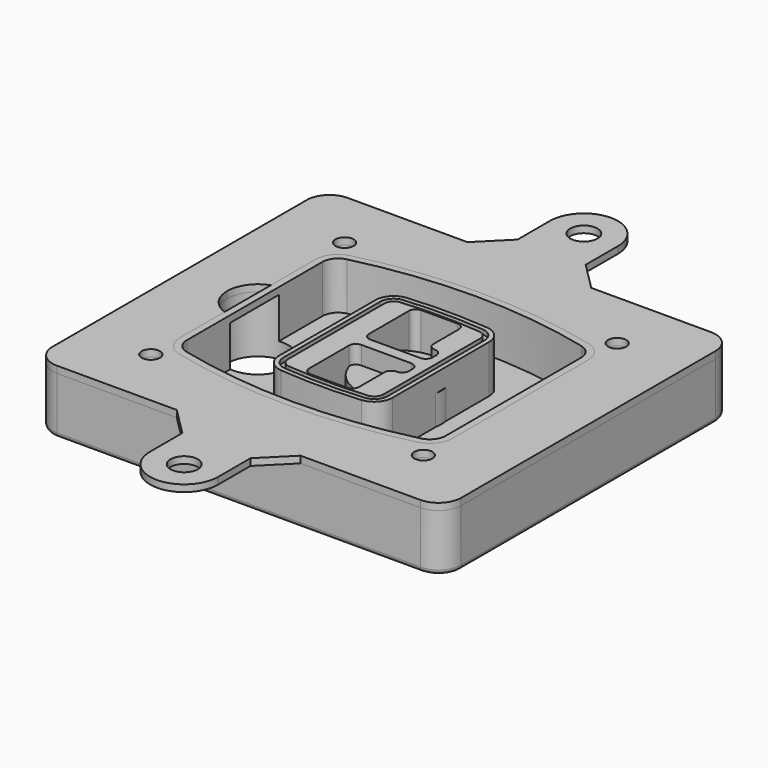
from build123d import *

# Parameters (mm, degrees)
F0_R      = 4
F1_DEPTH  = 25
F2_DEPTH  = 3
F3_DEPTH  = 18
F5_DEPTH  = 21
F6_DEPTH  = 2
F8_DEPTH  = 20
F9_DEPTH  = 16
F10_DEPTH = 25
F7_R      = 6
F7_R_2    = 4
F11_DEPTH = 6
F13_DEPTH = 9
F15_R     = 2
F16_R     = 6
F16_R_2   = 4
F17_DEPTH = 3


# Not quite as in the source:
# - a feature of the source that left no trace in its solid (it failed there, or was rolled back) is left out
# - a feature names something its author has since deleted; it is built from what else it names


with BuildPart() as f1:
    # F0 (on Top) → F1 (new body)
    with BuildSketch(Plane.XY):
        with BuildLine():
            ThreePointArc((-90, -70), (-87.0710678119, -77.0710678119), (-80, -80))
            Line((-80, -80), (80, -80))
            ThreePointArc((80, -80), (87.0710678119, -77.0710678119), (90, -70))
            Line((90, -70), (90, 70))
            ThreePointArc((90, 70), (87.0710678119, 77.0710678119), (80, 80))
            Line((80, 80), (-80, 80))
            ThreePointArc((-80, 80), (-87.0710678119, 77.0710678119), (-90, 70))
            Line((-90, 70), (-90, -70))
        make_face()
        with Locations((-60, -53.3333333333)):
            Circle(F0_R, mode=Mode.SUBTRACT)
        with Locations((60, -53.3333333333)):
            Circle(F0_R, mode=Mode.SUBTRACT)
        with Locations((-60, 53.3333333333)):
            Circle(F0_R, mode=Mode.SUBTRACT)
        with BuildLine():
            ThreePointArc((-64, 37.2990447398), (-61.0143011354, 45.9411029726), (-53.3306899286, 50.8970778549))
            ThreePointArc((-53.3306899286, 50.8970778549), (0, 57.3333333333), (53.3306899286, 50.8970778549))
            ThreePointArc((53.3306899286, 50.8970778549), (61.0143011354, 45.9411029726), (64, 37.2990447398))
            Line((64, 37.2990447398), (64, -37.2990447398))
            ThreePointArc((64, -37.2990447398), (61.0143011354, -45.9411029726), (53.3306899286, -50.8970778549))
            ThreePointArc((53.3306899286, -50.8970778549), (0, -57.3333333333), (-53.3306899286, -50.8970778549))
            ThreePointArc((-53.3306899286, -50.8970778549), (-61.0143011354, -45.9411029726), (-64, -37.2990447398))
            Line((-64, -37.2990447398), (-64, 37.2990447398))
        make_face(mode=Mode.SUBTRACT)
        with Locations((60, 53.3333333333)):
            Circle(F0_R, mode=Mode.SUBTRACT)
        with BuildLine():
            ThreePointArc((53.3306899286, 50.8970778549), (0, 57.3333333333), (-53.3306899286, 50.8970778549))
            ThreePointArc((-53.3306899286, 50.8970778549), (-61.0143011354, 45.9411029726), (-64, 37.2990447398))
            Line((-64, 37.2990447398), (-64, -37.2990447398))
            ThreePointArc((-64, -37.2990447398), (-61.0143011354, -45.9411029726), (-53.3306899286, -50.8970778549))
            ThreePointArc((-53.3306899286, -50.8970778549), (0, -57.3333333333), (53.3306899286, -50.8970778549))
            ThreePointArc((53.3306899286, -50.8970778549), (61.0143011354, -45.9411029726), (64, -37.2990447398))
            Line((64, -37.2990447398), (64, 37.2990447398))
            ThreePointArc((64, 37.2990447398), (61.0143011354, 45.9411029726), (53.3306899286, 50.8970778549))
        make_face()
        with BuildLine():
            Line((-60, -37.2990447398), (-60, 37.2990447398))
            ThreePointArc((-60, 37.2990447398), (-57.8673579538, 43.4719434775), (-52.3790642347, 47.0119255363))
            ThreePointArc((-52.3790642347, 47.0119255363), (0, 53.3333333333), (52.3790642347, 47.0119255363))
            ThreePointArc((52.3790642347, 47.0119255363), (57.8673579538, 43.4719434775), (60, 37.2990447398))
            Line((60, 37.2990447398), (60, -37.2990447398))
            ThreePointArc((60, -37.2990447398), (57.8673579538, -43.4719434775), (52.3790642347, -47.0119255363))
            ThreePointArc((52.3790642347, -47.0119255363), (0, -53.3333333333), (-52.3790642347, -47.0119255363))
            ThreePointArc((-52.3790642347, -47.0119255363), (-57.8673579538, -43.4719434775), (-60, -37.2990447398))
        make_face(mode=Mode.SUBTRACT)
        with BuildLine():
            ThreePointArc((-52.3790642347, 47.0119255363), (-57.8673579538, 43.4719434775), (-60, 37.2990447398))
            Line((-60, 37.2990447398), (-60, -37.2990447398))
            ThreePointArc((-60, -37.2990447398), (-57.8673579538, -43.4719434775), (-52.3790642347, -47.0119255363))
            ThreePointArc((-52.3790642347, -47.0119255363), (0, -53.3333333333), (52.3790642347, -47.0119255363))
            ThreePointArc((52.3790642347, -47.0119255363), (57.8673579538, -43.4719434775), (60, -37.2990447398))
            Line((60, -37.2990447398), (60, 37.2990447398))
            ThreePointArc((60, 37.2990447398), (57.8673579538, 43.4719434775), (52.3790642347, 47.0119255363))
            ThreePointArc((52.3790642347, 47.0119255363), (0, 53.3333333333), (-52.3790642347, 47.0119255363))
        make_face()
        with BuildLine():
            ThreePointArc((51.6653449643, 44.0980612973), (55.5071505677, 41.6200738562), (57, 37.2990447398))
            Line((57, 37.2990447398), (57, -37.2990447398))
            ThreePointArc((57, -37.2990447398), (55.5071505677, -41.6200738562), (51.6653449643, -44.0980612973))
            ThreePointArc((51.6653449643, -44.0980612973), (0, -50.3333333333), (-51.6653449643, -44.0980612973))
            ThreePointArc((-51.6653449643, -44.0980612973), (-55.5071505677, -41.6200738562), (-57, -37.2990447398))
            Line((-57, -37.2990447398), (-57, 37.2990447398))
            ThreePointArc((-57, 37.2990447398), (-55.5071505677, 41.6200738562), (-51.6653449643, 44.0980612973))
            ThreePointArc((-51.6653449643, 44.0980612973), (0, 50.3333333333), (51.6653449643, 44.0980612973))
        make_face(mode=Mode.SUBTRACT)
        with BuildLine():
            Line((57, -37.2990447398), (57, 37.2990447398))
            ThreePointArc((57, 37.2990447398), (55.5071505677, 41.6200738562), (51.6653449643, 44.0980612973))
            ThreePointArc((51.6653449643, 44.0980612973), (0, 50.3333333333), (-51.6653449643, 44.0980612973))
            ThreePointArc((-51.6653449643, 44.0980612973), (-55.5071505677, 41.6200738562), (-57, 37.2990447398))
            Line((-57, 37.2990447398), (-57, -37.2990447398))
            ThreePointArc((-57, -37.2990447398), (-55.5071505677, -41.6200738562), (-51.6653449643, -44.0980612973))
            ThreePointArc((-51.6653449643, -44.0980612973), (0, -50.3333333333), (51.6653449643, -44.0980612973))
            ThreePointArc((51.6653449643, -44.0980612973), (55.5071505677, -41.6200738562), (57, -37.2990447398))
        make_face()
    extrude(amount=-F1_DEPTH)

    # F0 (on Top) → F2 (join)
    with BuildSketch(Plane.XY):
        with BuildLine():
            ThreePointArc((-52.3790642347, 47.0119255363), (-57.8673579538, 43.4719434775), (-60, 37.2990447398))
            Line((-60, 37.2990447398), (-60, -37.2990447398))
            ThreePointArc((-60, -37.2990447398), (-57.8673579538, -43.4719434775), (-52.3790642347, -47.0119255363))
            ThreePointArc((-52.3790642347, -47.0119255363), (0, -53.3333333333), (52.3790642347, -47.0119255363))
            ThreePointArc((52.3790642347, -47.0119255363), (57.8673579538, -43.4719434775), (60, -37.2990447398))
            Line((60, -37.2990447398), (60, 37.2990447398))
            ThreePointArc((60, 37.2990447398), (57.8673579538, 43.4719434775), (52.3790642347, 47.0119255363))
            ThreePointArc((52.3790642347, 47.0119255363), (0, 53.3333333333), (-52.3790642347, 47.0119255363))
        make_face()
        with BuildLine():
            ThreePointArc((51.6653449643, 44.0980612973), (55.5071505677, 41.6200738562), (57, 37.2990447398))
            Line((57, 37.2990447398), (57, -37.2990447398))
            ThreePointArc((57, -37.2990447398), (55.5071505677, -41.6200738562), (51.6653449643, -44.0980612973))
            ThreePointArc((51.6653449643, -44.0980612973), (0, -50.3333333333), (-51.6653449643, -44.0980612973))
            ThreePointArc((-51.6653449643, -44.0980612973), (-55.5071505677, -41.6200738562), (-57, -37.2990447398))
            Line((-57, -37.2990447398), (-57, 37.2990447398))
            ThreePointArc((-57, 37.2990447398), (-55.5071505677, 41.6200738562), (-51.6653449643, 44.0980612973))
            ThreePointArc((-51.6653449643, 44.0980612973), (0, 50.3333333333), (51.6653449643, 44.0980612973))
        make_face(mode=Mode.SUBTRACT)
    extrude(amount=F2_DEPTH)

    # F0 (on Top) → F3 (cut)
    with BuildSketch(Plane.XY):
        with BuildLine():
            Line((57, -37.2990447398), (57, 37.2990447398))
            ThreePointArc((57, 37.2990447398), (55.5071505677, 41.6200738562), (51.6653449643, 44.0980612973))
            ThreePointArc((51.6653449643, 44.0980612973), (0, 50.3333333333), (-51.6653449643, 44.0980612973))
            ThreePointArc((-51.6653449643, 44.0980612973), (-55.5071505677, 41.6200738562), (-57, 37.2990447398))
            Line((-57, 37.2990447398), (-57, -37.2990447398))
            ThreePointArc((-57, -37.2990447398), (-55.5071505677, -41.6200738562), (-51.6653449643, -44.0980612973))
            ThreePointArc((-51.6653449643, -44.0980612973), (0, -50.3333333333), (51.6653449643, -44.0980612973))
            ThreePointArc((51.6653449643, -44.0980612973), (55.5071505677, -41.6200738562), (57, -37.2990447398))
        make_face()
    extrude(amount=-F3_DEPTH, mode=Mode.SUBTRACT)

    # F4 (on face) → F5 (join, through all)
    with BuildSketch(Plane.XY.offset(3)):
        with BuildLine():
            ThreePointArc((-25, -26.587695628), (-22.8992979869, -31.9912392117), (-17.7004291845, -34.5569740744))
            ThreePointArc((-17.7004291845, -34.5569740744), (0, -35.3333333333), (17.7004291845, -34.5569740744))
            ThreePointArc((17.7004291845, -34.5569740744), (22.8992979869, -31.9912392117), (25, -26.587695628))
            Line((25, -26.587695628), (25, 26.587695628))
            ThreePointArc((25, 26.587695628), (22.8992979869, 31.9912392117), (17.7004291845, 34.5569740744))
            ThreePointArc((17.7004291845, 34.5569740744), (0, 35.3333333333), (-17.7004291845, 34.5569740744))
            ThreePointArc((-17.7004291845, 34.5569740744), (-22.8992979869, 31.9912392117), (-25, 26.587695628))
            Line((-25, 26.587695628), (-25, -26.587695628))
        make_face()
        with BuildLine():
            ThreePointArc((17.5253218884, 32.5646544628), (21.4244734902, 30.6403533158), (23, 26.587695628))
            Line((23, 26.587695628), (23, -26.587695628))
            ThreePointArc((23, -26.587695628), (21.4244734902, -30.6403533158), (17.5253218884, -32.5646544628))
            ThreePointArc((17.5253218884, -32.5646544628), (0, -33.3333333333), (-17.5253218884, -32.5646544628))
            ThreePointArc((-17.5253218884, -32.5646544628), (-21.4244734902, -30.6403533158), (-23, -26.587695628))
            Line((-23, -26.587695628), (-23, 26.587695628))
            ThreePointArc((-23, 26.587695628), (-21.4244734902, 30.6403533158), (-17.5253218884, 32.5646544628))
            ThreePointArc((-17.5253218884, 32.5646544628), (0, 33.3333333333), (17.5253218884, 32.5646544628))
        make_face(mode=Mode.SUBTRACT)
        with BuildLine():
            Line((23, -26.587695628), (23, 26.587695628))
            ThreePointArc((23, 26.587695628), (21.4244734902, 30.6403533158), (17.5253218884, 32.5646544628))
            ThreePointArc((17.5253218884, 32.5646544628), (0, 33.3333333333), (-17.5253218884, 32.5646544628))
            ThreePointArc((-17.5253218884, 32.5646544628), (-21.4244734902, 30.6403533158), (-23, 26.587695628))
            Line((-23, 26.587695628), (-23, -26.587695628))
            ThreePointArc((-23, -26.587695628), (-21.4244734902, -30.6403533158), (-17.5253218884, -32.5646544628))
            ThreePointArc((-17.5253218884, -32.5646544628), (0, -33.3333333333), (17.5253218884, -32.5646544628))
            ThreePointArc((17.5253218884, -32.5646544628), (21.4244734902, -30.6403533158), (23, -26.587695628))
        make_face()
        with BuildLine():
            ThreePointArc((17.3502145923, 30.5723348512), (19.9496489934, 29.2894674198), (21, 26.587695628))
            Line((21, 26.587695628), (21, -26.587695628))
            ThreePointArc((21, -26.587695628), (19.9496489934, -29.2894674198), (17.3502145923, -30.5723348512))
            ThreePointArc((17.3502145923, -30.5723348512), (0, -31.3333333333), (-17.3502145923, -30.5723348512))
            ThreePointArc((-17.3502145923, -30.5723348512), (-19.9496489934, -29.2894674198), (-21, -26.587695628))
            Line((-21, -26.587695628), (-21, 26.587695628))
            ThreePointArc((-21, 26.587695628), (-19.9496489934, 29.2894674198), (-17.3502145923, 30.5723348512))
            ThreePointArc((-17.3502145923, 30.5723348512), (0, 31.3333333333), (17.3502145923, 30.5723348512))
        make_face(mode=Mode.SUBTRACT)
        with BuildLine():
            Line((21, -26.587695628), (21, 26.587695628))
            ThreePointArc((21, 26.587695628), (19.9496489934, 29.2894674198), (17.3502145923, 30.5723348512))
            ThreePointArc((17.3502145923, 30.5723348512), (0, 31.3333333333), (-17.3502145923, 30.5723348512))
            ThreePointArc((-17.3502145923, 30.5723348512), (-19.9496489934, 29.2894674198), (-21, 26.587695628))
            Line((-21, 26.587695628), (-21, -26.587695628))
            ThreePointArc((-21, -26.587695628), (-19.9496489934, -29.2894674198), (-17.3502145923, -30.5723348512))
            ThreePointArc((-17.3502145923, -30.5723348512), (0, -31.3333333333), (17.3502145923, -30.5723348512))
            ThreePointArc((17.3502145923, -30.5723348512), (19.9496489934, -29.2894674198), (21, -26.587695628))
        make_face()
        with BuildLine():
            Line((-8, -2.5), (14, -2.5))
            ThreePointArc((14, -2.5), (16.1213203436, -3.3786796564), (17, -5.5))
            Line((17, -5.5), (17, -7.5))
            ThreePointArc((17, -7.5), (16.1213203436, -9.6213203436), (14, -10.5))
            ThreePointArc((14, -10.5), (11.8786796564, -11.3786796564), (11, -13.5))
            Line((11, -13.5), (11, -27.5))
            ThreePointArc((11, -27.5), (10.1213203436, -29.6213203436), (8, -30.5))
            Line((8, -30.5), (-8, -30.5))
            ThreePointArc((-8, -30.5), (-10.1213203436, -29.6213203436), (-11, -27.5))
            Line((-11, -27.5), (-11, -5.5))
            ThreePointArc((-11, -5.5), (-10.1213203436, -3.3786796564), (-8, -2.5))
        make_face(mode=Mode.SUBTRACT)
        with BuildLine():
            ThreePointArc((-8, 2.5), (-10.1213203436, 3.3786796564), (-11, 5.5))
            Line((-11, 5.5), (-11, 27.5))
            ThreePointArc((-11, 27.5), (-10.1213203436, 29.6213203436), (-8, 30.5))
            Line((-8, 30.5), (8, 30.5))
            ThreePointArc((8, 30.5), (10.1213203436, 29.6213203436), (11, 27.5))
            Line((11, 27.5), (11, 13.5))
            ThreePointArc((11, 13.5), (11.8786796564, 11.3786796564), (14, 10.5))
            ThreePointArc((14, 10.5), (16.1213203436, 9.6213203436), (17, 7.5))
            Line((17, 7.5), (17, 5.5))
            ThreePointArc((17, 5.5), (16.1213203436, 3.3786796564), (14, 2.5))
            Line((14, 2.5), (-8, 2.5))
        make_face(mode=Mode.SUBTRACT)
    extrude(amount=-F5_DEPTH)

    # F4 (on face) → F6 (cut)
    with BuildSketch(Plane.XY.offset(3)):
        with BuildLine():
            Line((23, -26.587695628), (23, 26.587695628))
            ThreePointArc((23, 26.587695628), (21.4244734902, 30.6403533158), (17.5253218884, 32.5646544628))
            ThreePointArc((17.5253218884, 32.5646544628), (0, 33.3333333333), (-17.5253218884, 32.5646544628))
            ThreePointArc((-17.5253218884, 32.5646544628), (-21.4244734902, 30.6403533158), (-23, 26.587695628))
            Line((-23, 26.587695628), (-23, -26.587695628))
            ThreePointArc((-23, -26.587695628), (-21.4244734902, -30.6403533158), (-17.5253218884, -32.5646544628))
            ThreePointArc((-17.5253218884, -32.5646544628), (0, -33.3333333333), (17.5253218884, -32.5646544628))
            ThreePointArc((17.5253218884, -32.5646544628), (21.4244734902, -30.6403533158), (23, -26.587695628))
        make_face()
        with BuildLine():
            ThreePointArc((17.3502145923, 30.5723348512), (19.9496489934, 29.2894674198), (21, 26.587695628))
            Line((21, 26.587695628), (21, -26.587695628))
            ThreePointArc((21, -26.587695628), (19.9496489934, -29.2894674198), (17.3502145923, -30.5723348512))
            ThreePointArc((17.3502145923, -30.5723348512), (0, -31.3333333333), (-17.3502145923, -30.5723348512))
            ThreePointArc((-17.3502145923, -30.5723348512), (-19.9496489934, -29.2894674198), (-21, -26.587695628))
            Line((-21, -26.587695628), (-21, 26.587695628))
            ThreePointArc((-21, 26.587695628), (-19.9496489934, 29.2894674198), (-17.3502145923, 30.5723348512))
            ThreePointArc((-17.3502145923, 30.5723348512), (0, 31.3333333333), (17.3502145923, 30.5723348512))
        make_face(mode=Mode.SUBTRACT)
    extrude(amount=-F6_DEPTH, mode=Mode.SUBTRACT)

    # F7 (on face) → F8 (join)
    with BuildSketch(Plane(origin=(0, 0, -25), x_dir=(1, 0, 0), z_dir=(0, 0, -1))):
        with BuildLine():
            ThreePointArc((-6.71157564, 0), (6.7567035675, 13.4682792075), (20.224982775, 0))
            Line((20.224982775, 0), (25.224982775, 0))
            ThreePointArc((25.224982775, 0), (6.7567035675, 18.4682792075), (-11.71157564, 0))
            Line((-11.71157564, 0), (-6.71157564, 0))
        make_face()
        with BuildLine():
            Line((-6.71157564, 0), (20.224982775, 0))
            ThreePointArc((20.224982775, 0), (6.7567035675, 13.4682792075), (-6.71157564, 0))
        make_face()
        with BuildLine():
            ThreePointArc((-6.71157564, 0), (6.7567035675, -13.4682792075), (20.224982775, 0))
            Line((20.224982775, 0), (-6.71157564, 0))
        make_face()
        with BuildLine():
            Line((25.224982775, 0), (20.224982775, 0))
            ThreePointArc((20.224982775, 0), (6.7567035675, -13.4682792075), (-6.71157564, 0))
            Line((-6.71157564, 0), (-11.71157564, 0))
            ThreePointArc((-11.71157564, 0), (6.7567035675, -18.4682792075), (25.224982775, 0))
        make_face()
    extrude(amount=-F8_DEPTH)

    # F7 (on face) → F9 (cut)
    with BuildSketch(Plane(origin=(0, 0, -25), x_dir=(1, 0, 0), z_dir=(0, 0, -1))):
        with BuildLine():
            Line((-6.71157564, 0), (20.224982775, 0))
            ThreePointArc((20.224982775, 0), (6.7567035675, 13.4682792075), (-6.71157564, 0))
        make_face()
        with BuildLine():
            ThreePointArc((-6.71157564, 0), (6.7567035675, -13.4682792075), (20.224982775, 0))
            Line((20.224982775, 0), (-6.71157564, 0))
        make_face()
    extrude(amount=-F9_DEPTH, mode=Mode.SUBTRACT)

    # F7 (on face) → F10 (cut)
    with BuildSketch(Plane(origin=(0, 0, -25), x_dir=(1, 0, 0), z_dir=(0, 0, -1))):
        with BuildLine():
            Line((-69.0318229325, 0), (-42.0952645175, 0))
            ThreePointArc((-42.0952645175, 0), (-55.563543725, 13.4682792075), (-69.0318229325, 0))
        make_face()
        with BuildLine():
            ThreePointArc((-69.0318229325, 0), (-55.563543725, -13.4682792075), (-42.0952645175, 0))
            Line((-42.0952645175, 0), (-69.0318229325, 0))
        make_face()
    extrude(amount=-F10_DEPTH, mode=Mode.SUBTRACT)

    # F7 (on face) → F11 (cut)
    with BuildSketch(Plane(origin=(0, 0, -25), x_dir=(1, 0, 0), z_dir=(0, 0, -1))):
        with Locations((60, -53.3333333333)):
            Circle(F7_R)
        with Locations((60, -53.3333333333)):
            Circle(F7_R_2, mode=Mode.SUBTRACT)
        with Locations((-60, -53.3333333333)):
            Circle(F7_R)
        with Locations((-60, -53.3333333333)):
            Circle(F7_R_2, mode=Mode.SUBTRACT)
        with Locations((-60, 53.3333333333)):
            Circle(F7_R)
        with Locations((-60, 53.3333333333)):
            Circle(F7_R_2, mode=Mode.SUBTRACT)
        with Locations((60, 53.3333333333)):
            Circle(F7_R)
        with Locations((60, 53.3333333333)):
            Circle(F7_R_2, mode=Mode.SUBTRACT)
    extrude(amount=-F11_DEPTH, mode=Mode.SUBTRACT)

    # F12 (on face) → F13 (cut, through all)
    with BuildSketch(Plane(origin=(0, 0, -9), x_dir=(1, 0, 0), z_dir=(0, 0, -1))):
        with BuildLine():
            ThreePointArc((20.224982775, 0), (20.1663399806, 1.2554664788), (19.9909222755, 2.5))
            Line((19.9909222755, 2.5), (14, 2.5))
            ThreePointArc((14, 2.5), (16.1213203436, 3.3786796564), (17, 5.5))
            Line((17, 5.5), (17, 7.5))
            ThreePointArc((17, 7.5), (16.1213203436, 9.6213203436), (14, 10.5))
            ThreePointArc((14, 10.5), (12.1627255951, 11.1284134507), (11.0951631559, 12.750384826))
            ThreePointArc((11.0951631559, 12.750384826), (11.0476113807, 12.7664660322), (11, 12.7823698976))
            Line((11, 12.7823698976), (11, -12.7823698976))
            ThreePointArc((11, -12.7823698976), (11.0476113807, -12.7664660322), (11.0951631559, -12.750384826))
            ThreePointArc((11.0951631559, -12.750384826), (12.1627255951, -11.1284134507), (14, -10.5))
            ThreePointArc((14, -10.5), (16.1213203436, -9.6213203436), (17, -7.5))
            Line((17, -7.5), (17, -5.5))
            ThreePointArc((17, -5.5), (16.1213203436, -3.3786796564), (14, -2.5))
            Line((14, -2.5), (19.9909222755, -2.5))
            ThreePointArc((19.9909222755, -2.5), (20.1663399806, -1.2554664788), (20.224982775, 0))
        make_face()
    extrude(amount=F13_DEPTH, mode=Mode.SUBTRACT)

    # F15
    f15_edges = [f1.edges().sort_by_distance(p)[0] for p in [
        (0, -80, -25),
        (-87.071068, -77.071068, -25),
        (-90, 0, -25),
        (-87.071068, 77.071068, -25),
        (87.071068, -77.071068, -25),
        (0, 80, -25),
        (90, 0, -25),
        (87.071068, 77.071068, -25),
    ]]
    fillet(f15_edges, radius=F15_R)


with BuildPart() as f17:
    # F16 (on face) → F17 (new body, through all)
    with BuildSketch(Plane.XY):
        with BuildLine():
            Line((-27.25, 80), (27.25, 80))
            Line((27.25, 80), (15, 92.25))
            Line((15, 92.25), (15, 110))
            ThreePointArc((15, 110), (0, 125), (-15, 110))
            Line((-15, 110), (-15, 92.25))
            Line((-15, 92.25), (-27.25, 80))
        make_face()
        with Locations((0, 110)):
            Circle(F16_R, mode=Mode.SUBTRACT)
        with BuildLine():
            Line((15, -92.25), (27.25, -80))
            Line((27.25, -80), (-27.25, -80))
            Line((-27.25, -80), (-15, -92.25))
            Line((-15, -92.25), (-15, -110))
            ThreePointArc((-15, -110), (0, -125), (15, -110))
            Line((15, -110), (15, -92.25))
        make_face()
        with Locations((0, -110)):
            Circle(F16_R, mode=Mode.SUBTRACT)
        with BuildLine():
            ThreePointArc((80, -80), (87.0710678119, -77.0710678119), (90, -70))
            Line((90, -70), (90, 70))
            ThreePointArc((90, 70), (87.0710678119, 77.0710678119), (80, 80))
            Line((80, 80), (27.25, 80))
            Line((27.25, 80), (-27.25, 80))
            Line((-27.25, 80), (-80, 80))
            ThreePointArc((-80, 80), (-87.0710678119, 77.0710678119), (-90, 70))
            Line((-90, 70), (-90, -70))
            ThreePointArc((-90, -70), (-87.0710678119, -77.0710678119), (-80, -80))
            Line((-80, -80), (-27.25, -80))
            Line((-27.25, -80), (27.25, -80))
            Line((27.25, -80), (80, -80))
        make_face()
        with Locations((-60, -53.3333333333)):
            Circle(F16_R_2, mode=Mode.SUBTRACT)
        with Locations((60, -53.3333333333)):
            Circle(F16_R_2, mode=Mode.SUBTRACT)
        with Locations((-60, 53.3333333333)):
            Circle(F16_R_2, mode=Mode.SUBTRACT)
        with BuildLine():
            ThreePointArc((-52.3790642347, 47.0119255363), (0, 53.3333333333), (52.3790642347, 47.0119255363))
            ThreePointArc((52.3790642347, 47.0119255363), (57.8673579538, 43.4719434775), (60, 37.2990447398))
            Line((60, 37.2990447398), (60, -37.2990447398))
            ThreePointArc((60, -37.2990447398), (57.8673579538, -43.4719434775), (52.3790642347, -47.0119255363))
            ThreePointArc((52.3790642347, -47.0119255363), (0, -53.3333333333), (-52.3790642347, -47.0119255363))
            ThreePointArc((-52.3790642347, -47.0119255363), (-57.8673579538, -43.4719434775), (-60, -37.2990447398))
            Line((-60, -37.2990447398), (-60, -12.7166190685))
            ThreePointArc((-60, -12.7166190685), (-66.5441169481, -7.798817635), (-69.0318229325, 0))
            ThreePointArc((-69.0318229325, 0), (-66.5441169481, 7.798817635), (-60, 12.7166190685))
            Line((-60, 12.7166190685), (-60, 37.2990447398))
            ThreePointArc((-60, 37.2990447398), (-57.8673579538, 43.4719434775), (-52.3790642347, 47.0119255363))
        make_face(mode=Mode.SUBTRACT)
        with Locations((60, 53.3333333333)):
            Circle(F16_R_2, mode=Mode.SUBTRACT)
    extrude(amount=F17_DEPTH)


solid = Compound([f1.part, f17.part])
